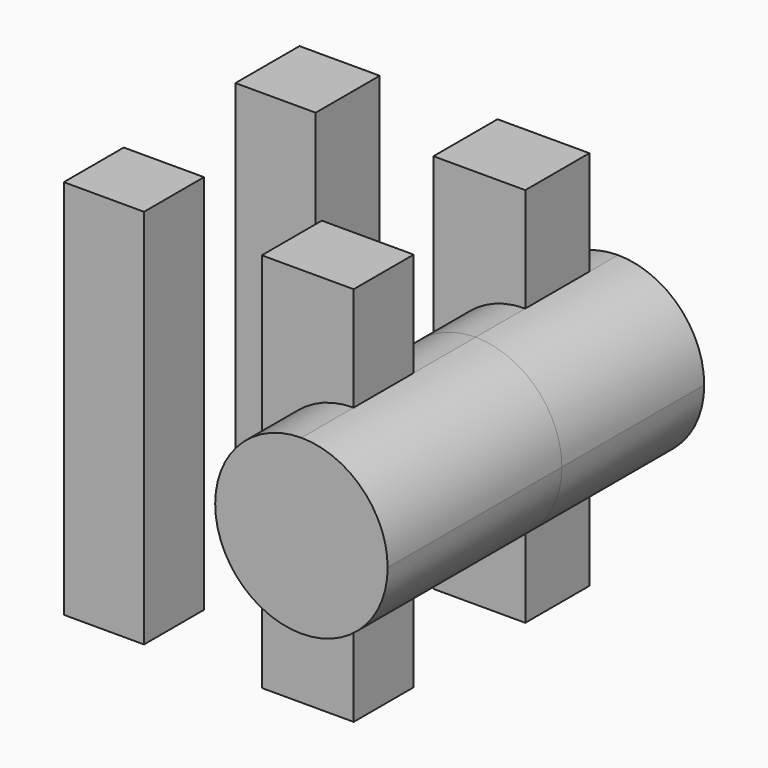
from build123d import *

# Parameters (mm, degrees)
F0_W          = 28.278099373
F0_H          = 28.2205780968
F1_DEPTH      = 134.2365369201
F0_W_2        = 32.3758274317
F0_H_2        = 26.4255460352
F3_DEPTH      = 62.7054031938
F3_DEPTH_BACK = 76.7472609878


with BuildPart() as f1:
    # F0 (on Top) → F1 (new body)
    with BuildSketch(Plane.XY):
        with Locations((-32.9155987129, 35.9918554313)):
            Rectangle(F0_W, F0_H)
    extrude(amount=F1_DEPTH)


with BuildPart() as f1b:
    # F0 (on Top) → F1, piece 2 (new body)
    with BuildSketch(Plane.XY):
        with Locations((38.9165617526, 35.9918554313)):
            Rectangle(F0_W_2, F0_H)
    extrude(amount=F1_DEPTH)


with BuildPart() as f1c:
    # F0 (on Top) → F1, piece 3 (new body)
    with BuildSketch(Plane.XY):
        with Locations((38.9165617526, -40.5146302655)):
            Rectangle(F0_W_2, F0_H_2)
    extrude(amount=F1_DEPTH)


with BuildPart() as f1d:
    # F0 (on Top) → F1, piece 4 (new body)
    with BuildSketch(Plane.XY):
        with Locations((-32.9155987129, -40.5146302655)):
            Rectangle(F0_W, F0_H_2)
    extrude(amount=F1_DEPTH)


with BuildPart() as f3:
    # F2 (on Front) → F3 (new body, two sides)
    with BuildSketch(Plane.XZ) as f3_sk:
        with BuildLine():
            ThreePointArc((85.4928173756, 67.11826846), (76.5922781, 88.6060710916), (55.1044754684, 97.5066103673))
            Line((55.1044754684, 97.5066103673), (55.1044754684, 36.7299265528))
            ThreePointArc((55.1044754684, 36.7299265528), (76.5922781, 45.6304658284), (85.4928173756, 67.11826846))
        make_face()
        with BuildLine():
            Line((55.1044754684, 36.7299265528), (55.1044754684, 97.5066103673))
            ThreePointArc((55.1044754684, 97.5066103673), (24.7161335612, 67.11826846), (55.1044754684, 36.7299265528))
        make_face()
    extrude(amount=-F3_DEPTH)
    extrude(f3_sk.sketch, amount=F3_DEPTH_BACK)


solid = Compound([f1.part, f1b.part, f1c.part, f1d.part, f3.part])
